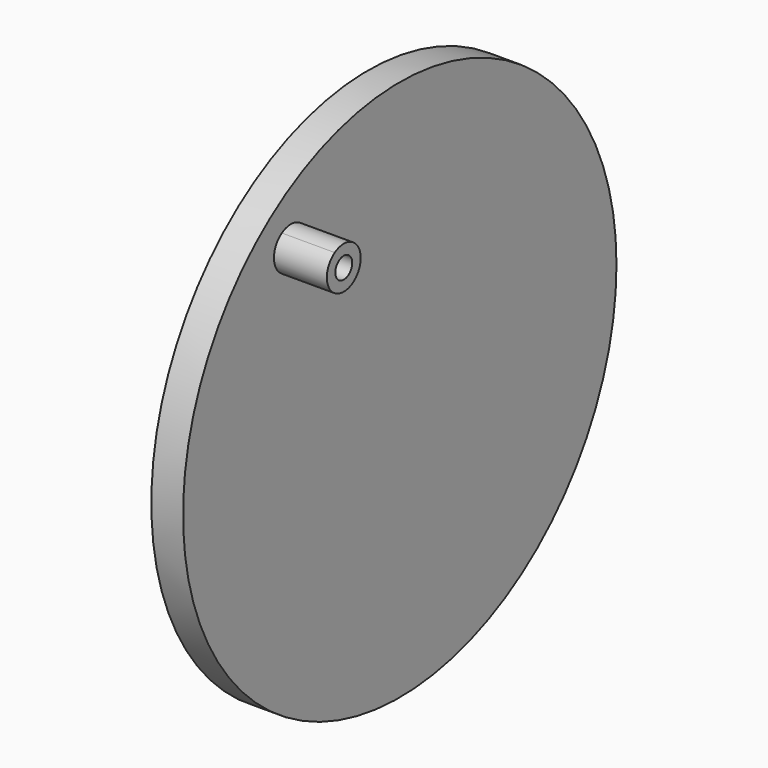
from build123d import *

# Parameters (mm, degrees)
F0_R     = 162.56
F1_DEPTH = 19.05
F4_DEPTH = 50.8
F7_T     = -6.35


# Not quite as in the source:
# - the program builds the solid bodies; features that only make, move or delete a surface that nothing else refers to are left out


with BuildPart() as f1:
    # F0 (on Right) → F1 (new body)
    with BuildSketch(Plane.YZ):
        Circle(F0_R)
    extrude(amount=F1_DEPTH)

    # F3 (on face) → F4 (join)
    with BuildSketch(Plane(origin=(0, 0, 0), x_dir=(0, -1, 0), z_dir=(-1, 0, 0))):
        with BuildLine():
            ThreePointArc((88.4545554599, 118.760558867), (78.8208582967, 120.384258227), (70.884610199, 114.6868476944))
            ThreePointArc((70.884610199, 114.6868476944), (84.557836343, 95.6406311102), (88.4545554599, 118.760558867))
        make_face()
    extrude(amount=-F4_DEPTH)

    # F7
    f7_openings = [f1.faces().sort_by_distance(p)[0] for p in [
        (50.8, -81.689347, 108.012445),
    ]]
    offset(amount=F7_T, openings=f7_openings, kind=Kind.INTERSECTION)


solid = f1.part
